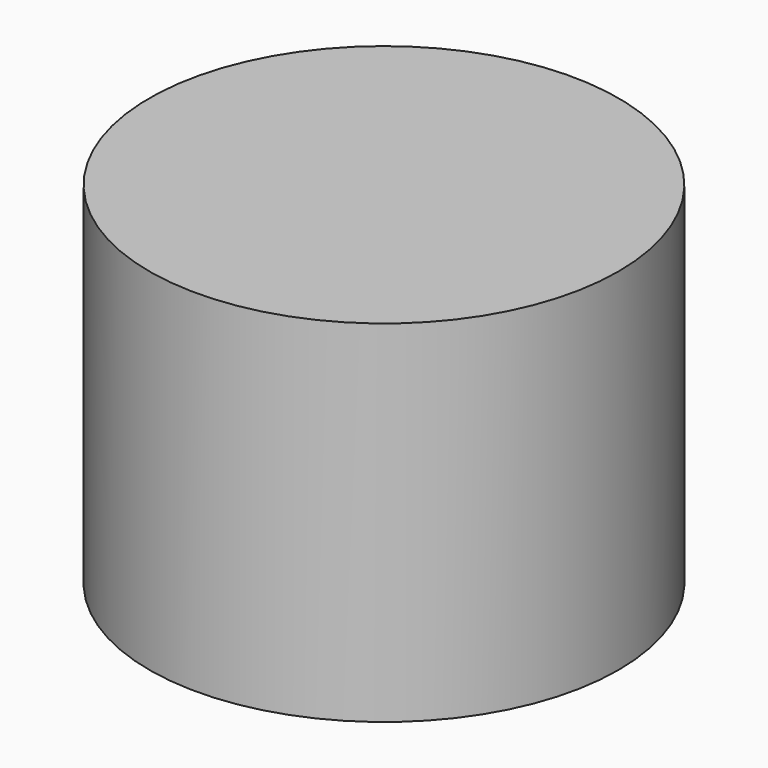
from build123d import *

# Parameters (mm, degrees)
F0_R     = 33.9631705584
F0_R_2   = 22.1322753086
F1_DEPTH = 25.4


# Not quite as in the source:
# - the program builds the solid bodies; features that only make, move or delete a surface that nothing else refers to are left out


with BuildPart() as f1:
    # F0 (on Top) → F1 (new body, symmetric)
    with BuildSketch(Plane.XY):
        with Locations((15.2396384771, -30.3521065738)):
            Circle(F0_R)
        with Locations((15.2396384771, -30.3521065738)):
            Circle(F0_R_2, mode=Mode.SUBTRACT)
        with Locations((15.2396384771, -30.3521065738)):
            Circle(F0_R_2)
    extrude(amount=F1_DEPTH, both=True)


solid = f1.part
